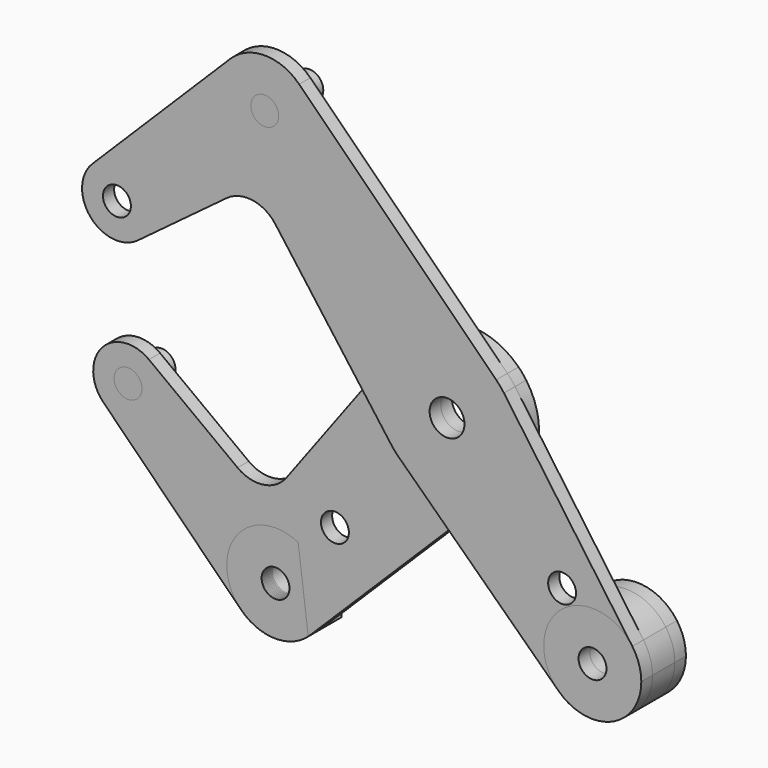
from build123d import *

# Parameters (mm, degrees)
F0_R     = 3.175
F0_R_2   = 3.96875
F1_DEPTH = 3.175
F2_DEPTH = 3.175
F4_R     = 3.175
F6_DEPTH = 9.525
F3_R     = 3.175


# Not quite as in the source:
# - a pattern or mirror of a feature is missing from the dataset's text; its kind, count and spacing are read off the source's solid


with BuildPart() as f1:
    # F0 (on Front) → F1 (new body)
    with BuildSketch(Plane.XZ):
        with BuildLine():
            ThreePointArc((14.7496603052, 14.7775566037), (26.3131341296, 21.1399199057), (38.6911584981, 16.5597336206))
            Line((38.6911584981, 16.5597336206), (-6.186140597, 61.2318347541))
            ThreePointArc((-6.186140597, 61.2318347541), (-3.7641062388, 57.6204552843), (-2.9133385399, 53.3561257439))
            ThreePointArc((-2.9133385399, 53.3561257439), (-18.2901680804, 43.0943934427), (-21.8655364829, 61.2318347541))
            Line((-21.8655364829, 61.2318347541), (-53.2879053781, 29.953142198))
            ThreePointArc((-53.2879053781, 29.953142198), (-44.6421714614, 31.6574445487), (-39.7506211331, 24.3276357622))
            ThreePointArc((-39.7506211331, 24.3276357622), (-40.5946025832, 20.7659085362), (-42.9470685869, 17.9616066227))
            Line((-42.9470685869, 17.9616066227), (-22.7062919024, 33.0357735381))
            ThreePointArc((-22.7062919024, 33.0357735381), (-16.8060800027, 34.5221488612), (-11.587003326, 31.3943619908))
            Line((-11.587003326, 31.3943619908), (7.72443139, 5.3239158017))
            Line((7.72443139, 5.3239158017), (14.7496603052, 14.7775566037))
        make_face()
        with BuildLine():
            ThreePointArc((52.9106217019, -41.2084486244), (53.372225282, -24.7793229574), (69.6857179674, -26.7791240605))
            Line((69.6857179674, -26.7791240605), (40.4443254491, 14.4870795127))
            ThreePointArc((40.4443254491, 14.4870795127), (42.6183923822, 10.124888825), (43.3665900081, 5.3087207489))
            ThreePointArc((43.3665900081, 5.3087207489), (42.1465203967, -0.7944456676), (38.6738479221, -5.9594970758))
            Line((38.6738479221, -5.9594970758), (27.6583771328, -16.8909360421))
            Line((27.6583771328, -16.8909360421), (52.9106217019, -41.2084486244))
        make_face()
        with Locations((53.6926918641, -20.310522387)):
            Circle(F0_R, mode=Mode.SUBTRACT)
        with BuildLine():
            ThreePointArc((-2.9133385399, 53.3561257439), (-3.7641062388, 57.6204552843), (-6.186140597, 61.2318347541))
            ThreePointArc((-6.186140597, 61.2318347541), (-14.0258385399, 64.4686257439), (-21.8655364829, 61.2318347541))
            ThreePointArc((-21.8655364829, 61.2318347541), (-18.2901680804, 43.0943934427), (-2.9133385399, 53.3561257439))
        make_face()
        with Locations((-14.0258385399, 53.3561257439)):
            Circle(F0_R, mode=Mode.SUBTRACT)
        with BuildLine():
            ThreePointArc((-39.7506211331, 24.3276357622), (-44.6421714614, 31.6574445487), (-53.2879053781, 29.953142198))
            ThreePointArc((-53.2879053781, 29.953142198), (-53.6992430247, 19.1439768369), (-42.9470685869, 17.9616066227))
            ThreePointArc((-42.9470685869, 17.9616066227), (-40.5946025832, 20.7659085362), (-39.7506211331, 24.3276357622))
        make_face()
        with Locations((-47.6881211331, 24.3276357622)):
            Circle(F0_R, mode=Mode.SUBTRACT)
        with BuildLine():
            ThreePointArc((52.9106217019, -41.2084486244), (64.9679691599, -43.4300404866), (71.7313031587, -33.2039751952))
            ThreePointArc((71.7313031587, -33.2039751952), (71.2075648205, -29.8326575419), (69.6857179674, -26.7791240605))
            ThreePointArc((69.6857179674, -26.7791240605), (53.372225282, -24.7793229574), (52.9106217019, -41.2084486244))
        make_face()
        with Locations((60.6188031587, -33.2039751952)):
            Circle(F0_R, mode=Mode.SUBTRACT)
        with BuildLine():
            ThreePointArc((43.3665900081, 5.3087207489), (42.6183923822, 10.124888825), (40.4443254491, 14.4870795127))
            ThreePointArc((40.4443254491, 14.4870795127), (39.6121271272, 15.5609500159), (38.6911584981, 16.5597336206))
            ThreePointArc((38.6911584981, 16.5597336206), (26.3131341296, 21.1399199057), (14.7496603052, 14.7775566037))
            ThreePointArc((14.7496603052, 14.7775566037), (11.6165946984, 5.3209238883), (14.7351179476, -4.1405144355))
            ThreePointArc((14.7351179476, -4.1405144355), (15.5661074803, -5.1697567874), (16.4799022127, -6.1262412929))
            ThreePointArc((16.4799022127, -6.1262412929), (27.6108563061, -10.5658312306), (38.6738479221, -5.9594970758))
            ThreePointArc((38.6738479221, -5.9594970758), (42.1465203967, -0.7944456676), (43.3665900081, 5.3087207489))
        make_face()
        with Locations((27.4915900081, 5.3087207489)):
            Circle(F0_R_2, mode=Mode.SUBTRACT)
        with BuildLine():
            ThreePointArc((14.7351179476, -4.1405144355), (11.6165946984, 5.3209238883), (14.7496603052, 14.7775566037))
            Line((14.7496603052, 14.7775566037), (7.72443139, 5.3239158017))
            Line((7.72443139, 5.3239158017), (14.7351179476, -4.1405144355))
        make_face()
        with BuildLine():
            Line((16.4799022127, -6.1262412929), (27.6583771328, -16.8909360421))
            Line((27.6583771328, -16.8909360421), (38.6738479221, -5.9594970758))
            ThreePointArc((38.6738479221, -5.9594970758), (27.6108563061, -10.5658312306), (16.4799022127, -6.1262412929))
        make_face()
    extrude(amount=F1_DEPTH)


with BuildPart() as f2:
    # F0 (on Front) → F2 (new body)
    with BuildSketch(Plane.XZ):
        with BuildLine():
            ThreePointArc((-21.9593287693, -50.530575103), (-14.1223086093, -53.7872753618), (-6.2720771563, -50.5625509241))
            ThreePointArc((-6.2720771563, -50.5625509241), (-3.8412064241, -46.9470149384), (-2.9871576961, -42.6747984468))
            ThreePointArc((-2.9871576961, -42.6747984468), (-18.3509552303, -32.4076603098), (-21.9593287693, -50.530575103))
        make_face()
        with Locations((-14.0996576961, -42.6747984468)):
            Circle(F0_R, mode=Mode.SUBTRACT)
        with BuildLine():
            ThreePointArc((-42.9309189236, -7.2069551619), (-53.6860610326, -8.3620190908), (-53.3021718997, -19.172194094))
            ThreePointArc((-53.3021718997, -19.172194094), (-44.6514800372, -20.8945951518), (-39.7506211331, -13.5609250539))
            ThreePointArc((-39.7506211331, -13.5609250539), (-40.5900862364, -10.0082068191), (-42.9309189236, -7.2069551619))
        make_face()
        with Locations((-47.6881211331, -13.5609250539)):
            Circle(F0_R, mode=Mode.SUBTRACT)
        with BuildLine():
            Line((16.4799022127, -6.1262412929), (27.6583771328, -16.8909360421))
            Line((27.6583771328, -16.8909360421), (38.6738479221, -5.9594970758))
            ThreePointArc((38.6738479221, -5.9594970758), (27.6108563061, -10.5658312306), (16.4799022127, -6.1262412929))
        make_face()
        with BuildLine():
            ThreePointArc((43.3665900081, 5.3087207489), (42.6183923822, 10.124888825), (40.4443254491, 14.4870795127))
            ThreePointArc((40.4443254491, 14.4870795127), (39.6121271272, 15.5609500159), (38.6911584981, 16.5597336206))
            ThreePointArc((38.6911584981, 16.5597336206), (26.3131341296, 21.1399199057), (14.7496603052, 14.7775566037))
            ThreePointArc((14.7496603052, 14.7775566037), (11.6165946984, 5.3209238883), (14.7351179476, -4.1405144355))
            ThreePointArc((14.7351179476, -4.1405144355), (15.5661074803, -5.1697567874), (16.4799022127, -6.1262412929))
            ThreePointArc((16.4799022127, -6.1262412929), (27.6108563061, -10.5658312306), (38.6738479221, -5.9594970758))
            ThreePointArc((38.6738479221, -5.9594970758), (42.1465203967, -0.7944456676), (43.3665900081, 5.3087207489))
        make_face()
        with Locations((27.4915900081, 5.3087207489)):
            Circle(F0_R_2, mode=Mode.SUBTRACT)
        with BuildLine():
            Line((-6.2720771563, -50.5625509241), (27.6583771328, -16.8909360421))
            Line((27.6583771328, -16.8909360421), (16.4799022127, -6.1262412929))
            ThreePointArc((16.4799022127, -6.1262412929), (15.5661074803, -5.1697567874), (14.7351179476, -4.1405144355))
            Line((14.7351179476, -4.1405144355), (7.72443139, 5.3239158017))
            Line((7.72443139, 5.3239158017), (-11.6156424823, -20.7014441798))
            ThreePointArc((-11.6156424823, -20.7014441798), (-16.8434561593, -23.8217771487), (-22.7438095433, -22.3209961443))
            Line((-22.7438095433, -22.3209961443), (-42.9309189236, -7.2069551619))
            ThreePointArc((-42.9309189236, -7.2069551619), (-40.5900862364, -10.0082068191), (-39.7506211331, -13.5609250539))
            ThreePointArc((-39.7506211331, -13.5609250539), (-44.6514800372, -20.8945951518), (-53.3021718997, -19.172194094))
            Line((-53.3021718997, -19.172194094), (-21.9593287693, -50.530575103))
            ThreePointArc((-21.9593287693, -50.530575103), (-18.3509552303, -32.4076603098), (-2.9871576961, -42.6747984468))
            ThreePointArc((-2.9871576961, -42.6747984468), (-3.8412064241, -46.9470149384), (-6.2720771563, -50.5625509241))
        make_face()
        with Locations((-0.5825021922, -27.0801547082)):
            Circle(F0_R, mode=Mode.SUBTRACT)
        with BuildLine():
            ThreePointArc((14.7351179476, -4.1405144355), (11.6165946984, 5.3209238883), (14.7496603052, 14.7775566037))
            Line((14.7496603052, 14.7775566037), (7.72443139, 5.3239158017))
            Line((7.72443139, 5.3239158017), (14.7351179476, -4.1405144355))
        make_face()
    extrude(amount=-F2_DEPTH)


with BuildPart() as f6:
    # F4 (on face) → F6 (new body, through all)
    with BuildSketch(Plane.XZ):
        with Locations((-47.6881211331, -13.5609250539)):
            Circle(F4_R)
    extrude(amount=-F6_DEPTH)


with BuildPart() as f6b:
    # F4 (on face) → F6, piece 2 (new body, through all)
    with BuildSketch(Plane.XZ):
        with BuildLine():
            Line((-7.8000620823, -41.876302922), (-8.9468139737, -32.8291975092))
            ThreePointArc((-8.9468139737, -32.8291975092), (-23.0532279759, -36.0929115218), (-21.9593287693, -50.530575103))
            ThreePointArc((-21.9593287693, -50.530575103), (-14.3847692181, -53.7836403158), (-6.653310191, -50.9234083348))
            Line((-6.653310191, -50.9234083348), (-7.8000620823, -41.876302922))
        make_face()
        with BuildLine():
            ThreePointArc((-10.9246576961, -42.6747984468), (-17.2683508839, -42.8748196497), (-10.9498598892, -42.2755506844))
            ThreePointArc((-10.9498598892, -42.2755506844), (-10.9309645083, -42.474777244), (-10.9246576961, -42.6747984468))
        make_face(mode=Mode.SUBTRACT)
    extrude(amount=-F6_DEPTH)


with BuildPart() as f6c:
    # F3 (on face) → F6, piece 3 (new body, through all)
    with BuildSketch(Plane.XZ.offset(3.175)):
        with BuildLine():
            ThreePointArc((52.9106217019, -41.2084486244), (64.9679691599, -43.4300404866), (71.7313031587, -33.2039751952))
            ThreePointArc((71.7313031587, -33.2039751952), (71.2075648205, -29.8326575419), (69.6857179674, -26.7791240605))
            ThreePointArc((69.6857179674, -26.7791240605), (53.372225282, -24.7793229574), (52.9106217019, -41.2084486244))
        make_face()
        with Locations((60.6188031587, -33.2039751952)):
            Circle(F3_R, mode=Mode.SUBTRACT)
    extrude(amount=-F6_DEPTH)

    # F6_3_copies: F6c across plane


with BuildPart() as f6d:
    # F3 (on face) → F6, piece 4 (new body, through all)
    with BuildSketch(Plane.XZ.offset(3.175)):
        with Locations((-14.0258385399, 53.3561257439)):
            Circle(F3_R)
    extrude(amount=-F6_DEPTH)

    # F6_4_copies: F6d across plane


with BuildPart() as f6c_1:
    add(f6c.part)
    add(f6c.part.mirror(Plane.ZX.offset(3.175)))


with BuildPart() as f6d_1:
    add(f6d.part)
    add(f6d.part.mirror(Plane.ZX.offset(3.175)))


solid = Compound([f1.part, f2.part, f6.part, f6b.part, f6c_1.part, f6d_1.part])
